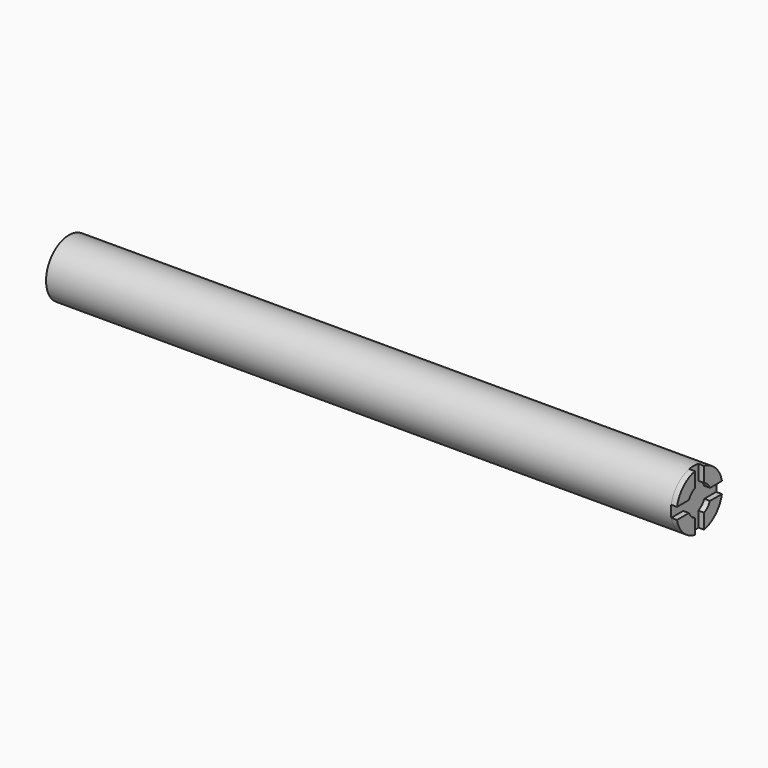
from build123d import *

# Parameters (mm, degrees)
F0_R     = 12.7
F1_DEPTH = 276.86
F3_DEPTH = 2.54


# Not quite as in the source:
# - after a boolean that leaves OpenCascade's solid faulty, fix() repairs it


with BuildPart() as f1:
    # F0 (on Right) → F1 (new body)
    with BuildSketch(Plane.YZ):
        Circle(F0_R)
    extrude(amount=-F1_DEPTH)

    # F2 (on face) → F3 (join)
    with BuildSketch(Plane.YZ):
        with BuildLine():
            ThreePointArc((-5.8198711326, 2.54), (-4.4901280605, 4.4901280605), (-2.54, 5.8198711326))
            Line((-2.54, 5.8198711326), (-2.54, 12.4434078933))
            ThreePointArc((-2.54, 12.4434078933), (-8.9802561211, 8.9802561211), (-12.4434078933, 2.54))
            Line((-12.4434078933, 2.54), (-5.8198711326, 2.54))
        make_face()
        with BuildLine():
            ThreePointArc((2.54, 5.8198711326), (4.4901280605, 4.4901280605), (5.8198711326, 2.54))
            Line((5.8198711326, 2.54), (12.4434078933, 2.54))
            ThreePointArc((12.4434078933, 2.54), (8.9802561211, 8.9802561211), (2.54, 12.4434078933))
            Line((2.54, 12.4434078933), (2.54, 5.8198711326))
        make_face()
        with BuildLine():
            Line((12.4434078933, -2.54), (5.8198711326, -2.54))
            ThreePointArc((5.8198711326, -2.54), (4.4901280605, -4.4901280605), (2.54, -5.8198711326))
            Line((2.54, -5.8198711326), (2.54, -12.4434078933))
            ThreePointArc((2.54, -12.4434078933), (8.9802561211, -8.9802561211), (12.4434078933, -2.54))
        make_face()
        with BuildLine():
            Line((-2.54, -12.4434078933), (-2.54, -5.8198711326))
            ThreePointArc((-2.54, -5.8198711326), (-4.4901280605, -4.4901280605), (-5.8198711326, -2.54))
            Line((-5.8198711326, -2.54), (-12.4434078933, -2.54))
            ThreePointArc((-12.4434078933, -2.54), (-8.9802561211, -8.9802561211), (-2.54, -12.4434078933))
        make_face()
    extrude(amount=F3_DEPTH)

    add(f1.part.fix(), mode=Mode.REPLACE)


solid = f1.part
